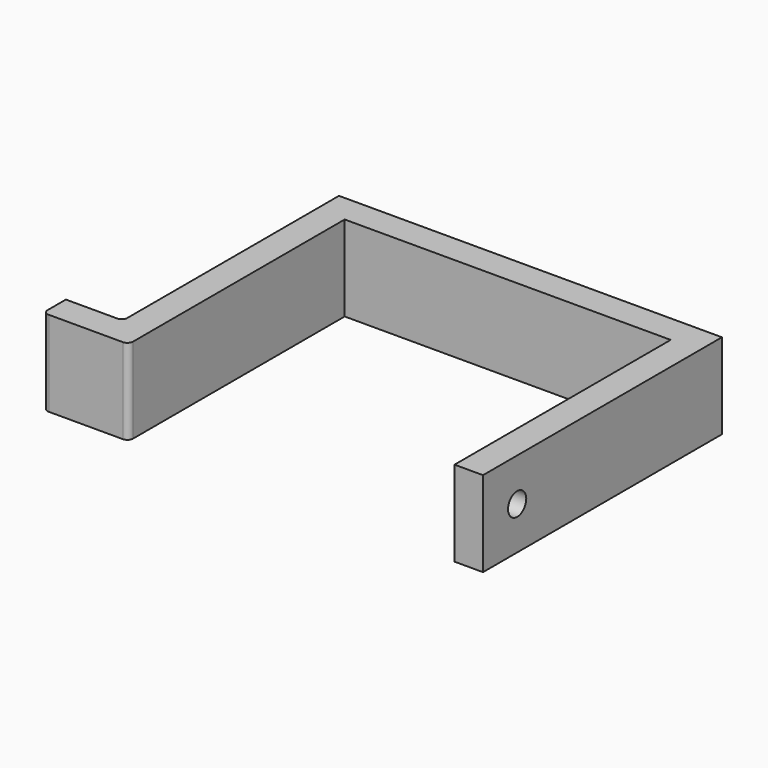
from build123d import *

# Parameters (mm, degrees)
F1_DEPTH  = 15
F2_R      = 2.325
F3_DEPTH  = 1.95
F4_R      = 4
F5_DEPTH  = 2
F6_W      = 0.2
F6_H      = 4.65
F7_REACH  = 19.6552990879
F8_R      = 1
F9_R      = 2
F10_DEPTH = 5


with BuildPart() as f1:
    # F0 (on Top) → F1 (new body)
    with BuildSketch(Plane.XY):
        Polygon((0, 0), (0, 20.15), (57.25, 20.15), (57.25, -27.3), (62.25, -27.3), (62.25, 25.15), (-5, 25.15), (-5, 0), (-5, -22.3), (-15, -22.3), (-15, -27.3), (0, -27.3), (0, -22.3), align=None)
    extrude(amount=F1_DEPTH)

    # F2 (on face) → F3 (join)
    with BuildSketch(Plane(origin=(-5, 0, 0), x_dir=(0, -1, 0), z_dir=(-1, 0, 0))):
        with Locations((-4.4213766232, 7.5)):
            Circle(F2_R)
        with BuildLine():
            ThreePointArc((-2.0963766232, 6.5151142198), (-4.4213766232, 4.975), (-6.7463766232, 6.5151142198))
            Line((-6.7463766232, 6.5151142198), (-6.7463766232, 0))
            Line((-6.7463766232, 0), (-2.0963766232, 0))
            Line((-2.0963766232, 0), (-2.0963766232, 6.5151142198))
        make_face()
    extrude(amount=F3_DEPTH)

    # F4 (on face) → F5 (join)
    with BuildSketch(Plane(origin=(-6.95, 0, 0), x_dir=(0, -1, 0), z_dir=(-1, 0, 0))):
        with Locations((-4.4213766232, 7.5)):
            Circle(F4_R)
        with BuildLine():
            ThreePointArc((-0.4213766232, 6.2193751525), (-4.4213766232, 3.3), (-8.4213766232, 6.2193751525))
            Line((-8.4213766232, 6.2193751525), (-8.4213766232, 0))
            Line((-8.4213766232, 0), (-0.4213766232, 0))
            Line((-0.4213766232, 0), (-0.4213766232, 6.2193751525))
        make_face()
    extrude(amount=F5_DEPTH)

    f7_end = f1.faces().sort_by_distance((-5.975, 4.4213766232, 4.975))[0]
    # F6 (on face) → F7 (cut, up to a face of the model that its end follows)
    with BuildSketch(Plane(origin=(0, 0, 0), x_dir=(1, 0, 0), z_dir=(0, 0, -1))):
        with Locations((-5.1, -4.4213766232)):
            Rectangle(F6_W, F6_H)
        with Locations((-6.85, -4.4213766232)):
            Rectangle(F6_W, F6_H)
    f7_long = extrude(amount=-F7_REACH, mode=Mode.PRIVATE)
    add(split(f7_long, bisect_by=f7_end, keep=Keep.BOTTOM, mode=Mode.PRIVATE), mode=Mode.SUBTRACT)

    # F8
    f8_edges = [f1.edges().sort_by_distance(p)[0] for p in [
        (-5, -22.3, 7.5),
        (0, -27.3, 7.5),
        (-15, -27.3, 7.5),
    ]]
    fillet(f8_edges, radius=F8_R)

    # F9 (on face) → F10 (cut, through all)
    with BuildSketch(Plane.YZ.offset(62.25)):
        with Locations((-19.8, 7.5)):
            Circle(F9_R)
    extrude(amount=-F10_DEPTH, mode=Mode.SUBTRACT)


solid = f1.part
